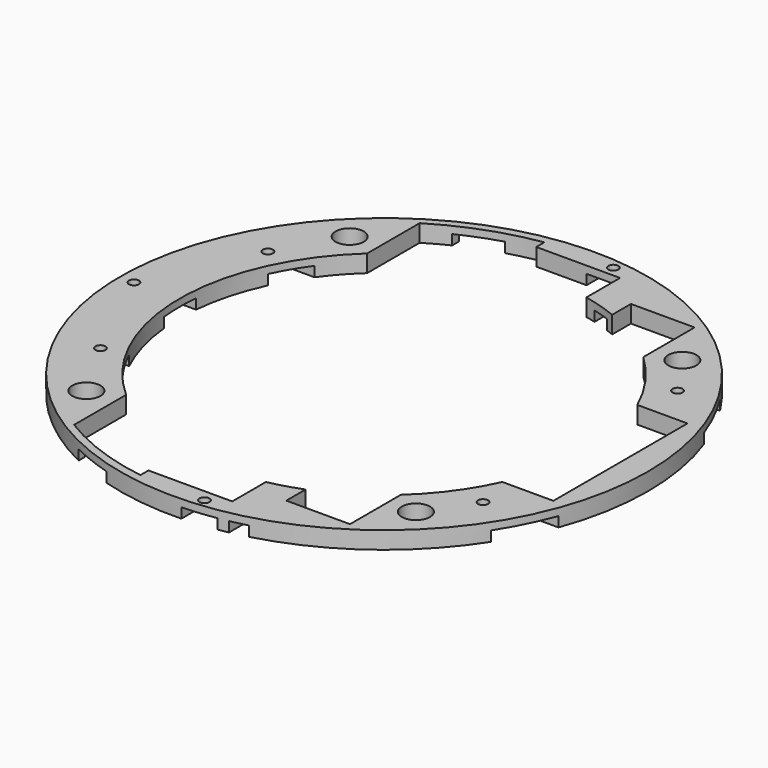
from build123d import *

# Parameters (mm, degrees)
F0_R     = 78.74
F0_R_2   = 4.208
F0_R_3   = 4.2080161266
F1_DEPTH = 5.17
F3_DEPTH = 3
F4_R     = 1.5
F5_DEPTH = 25


# Not quite as in the source:
# - a feature names something its author has since deleted; it is built from what else it names


with BuildPart() as f1:
    # F0 (on Top) → F1 (new body)
    with BuildSketch(Plane.XY):
        with Locations((-0.1257307514, 0.2739626218)):
            Circle(F0_R)
        with Locations((-49.0250116127, -49.6047185081)):
            Circle(F0_R_2, mode=Mode.SUBTRACT)
        with Locations((49.0554707364, -49.3247707953)):
            Circle(F0_R_3, mode=Mode.SUBTRACT)
        with Locations((-49.7306512766, 49.450932452)):
            Circle(F0_R_2, mode=Mode.SUBTRACT)
        with BuildLine():
            ThreePointArc((41.6625381497, 44.7120159348), (49.6362217188, 35.5549502263), (55.6382636856, 25))
            Line((55.6382636856, 25), (70.6142692486, 25))
            Line((70.6142692486, 25), (70.6142692486, -25))
            Line((70.6142692486, -25), (55.3920755218, -25))
            ThreePointArc((55.3920755218, -25), (49.182592498, -35.6382812281), (40.9624707364, -44.8121738117))
            Line((40.9624707364, -44.8121738117), (40.9624707364, -63.790228106))
            Line((40.9624707364, -63.790228106), (21.9624707364, -63.790228106))
            Line((21.9624707364, -63.790228106), (21.9624707364, -56.5864924857))
            ThreePointArc((21.9624707364, -56.5864924857), (17.2267771251, -58.2058669812), (12.3742692486, -59.4315647605))
            Line((12.3742692486, -59.4315647605), (12.3742692486, -71.9660373782))
            Line((12.3742692486, -71.9660373782), (-12.6257307514, -71.9660373782))
            Line((-12.6257307514, -71.9660373782), (-12.6257307514, -74.9675166541))
            ThreePointArc((-12.6257307514, -74.9675166541), (-27.09160778, -71.308076376), (-40.5250116127, -64.8121728344))
            Line((-40.5250116127, -64.8121728344), (-40.5250116127, -45.4305022137))
            ThreePointArc((-40.5250116127, -45.4305022137), (-61.1238878157, -0.2002048119), (-41.2306512766, 45.3448568731))
            Line((-41.2306512766, 45.3448568731), (-41.2306512766, 64.9332740284))
            ThreePointArc((-41.2306512766, 64.9332740284), (-27.3884909599, 71.6521165865), (-12.5, 75.5355537871))
            Line((-12.5, 75.5355537871), (-12.5, 72.5138622393))
            Line((-12.5, 72.5138622393), (0, 72.5138622393))
            Line((0, 72.5138622393), (12.5, 72.5138622393))
            Line((12.5, 72.5138622393), (12.5, 59.9530286583))
            ThreePointArc((12.5, 59.9530286583), (17.6487859305, 58.6269107626), (22.6625381497, 56.8574831953))
            Line((22.6625381497, 56.8574831953), (22.6625381497, 63.8574831953))
            Line((22.6625381497, 63.8574831953), (41.6625381497, 63.8574831953))
            Line((41.6625381497, 63.8574831953), (41.6625381497, 44.7120159348))
        make_face(mode=Mode.SUBTRACT)
        with Locations((49.75511293, 49.1690173001)):
            Circle(F0_R_2, mode=Mode.SUBTRACT)
    extrude(amount=F1_DEPTH)

    # F2 (on face) → F3 (cut)
    with BuildSketch(Plane(origin=(0, 0, 0), x_dir=(1, 0, 0), z_dir=(0, 0, -1))):
        with BuildLine():
            ThreePointArc((-22.6257307514, 75.1828965761), (-28.7215245435, 73.0899806842), (-34.6257307514, 70.5055372352))
            Line((-34.6257307514, 70.5055372352), (-34.6257307514, 68.081065471))
            ThreePointArc((-34.6257307514, 68.081065471), (-28.7284061022, 70.69020135), (-22.6257307514, 72.7742794712))
            Line((-22.6257307514, 72.7742794712), (-22.6257307514, 75.1828965761))
        make_face()
        with BuildLine():
            Line((-34.5, -68.6212157755), (-34.5, -71.1146092424))
            ThreePointArc((-34.5, -71.1146092424), (-28.5952430236, -73.6870028189), (-22.5, -75.7681986639))
            Line((-22.5, -75.7681986639), (-22.5, -73.2755617719))
            ThreePointArc((-22.5, -73.2755617719), (-28.595756362, -71.1952712241), (-34.5, -68.6212157755))
        make_face()
        with BuildLine():
            ThreePointArc((-49.5286609465, -36.0559481471), (-52.707319331, -31.1960670528), (-55.4094464584, -26.0559481471))
            Line((-55.4094464584, -26.0559481471), (-74.5251717599, -26.0559481471))
            ThreePointArc((-74.5251717599, -26.0559481471), (-72.5682702123, -31.1295306193), (-70.2658555864, -36.0559481471))
            Line((-70.2658555864, -36.0559481471), (-49.5286609465, -36.0559481471))
        make_face()
        with BuildLine():
            ThreePointArc((-60.8510849569, -6.0559481471), (-61.1253373513, -0.0548857934), (-60.807987598, 5.9440518529))
            Line((-60.807987598, 5.9440518529), (-78.6198317781, 5.9440518529))
            ThreePointArc((-78.6198317781, 5.9440518529), (-78.86542717, -0.0553124259), (-78.6531542631, -6.0559481471))
            Line((-78.6531542631, -6.0559481471), (-60.8510849569, -6.0559481471))
        make_face()
        with BuildLine():
            ThreePointArc((-55.2039997602, 25.9440518529), (-52.4464078958, 31.0875861785), (-49.2098975215, 35.9440518529))
            Line((-49.2098975215, 35.9440518529), (-70.0417019419, 35.9440518529))
            ThreePointArc((-70.0417019419, 35.9440518529), (-72.3803771023, 31.0190666452), (-74.3726385456, 25.9440518529))
            Line((-74.3726385456, 25.9440518529), (-55.2039997602, 25.9440518529))
        make_face()
        with BuildLine():
            Line((2.5, -72.5138622393), (2.5, -78.9701705229))
            ThreePointArc((2.5, -78.9701705229), (7.5155682015, -78.6423117834), (12.5, -77.9951214075))
            Line((12.5, -77.9951214075), (12.5, -72.5138622393))
            Line((12.5, -72.5138622393), (2.5, -72.5138622393))
        make_face()
        with BuildLine():
            ThreePointArc((12.3742692486, 77.4675166541), (7.3895759923, 78.1065691737), (2.3742692486, 78.4263397919))
            Line((2.3742692486, 78.4263397919), (2.3742692486, 71.9660373782))
            Line((2.3742692486, 71.9660373782), (12.3742692486, 71.9660373782))
            Line((12.3742692486, 71.9660373782), (12.3742692486, 77.4675166541))
        make_face()
        with BuildLine():
            ThreePointArc((20.3742692486, 75.7506228753), (17.8838503139, 76.3787776414), (15.3742692486, 76.9253741629))
            Line((15.3742692486, 76.9253741629), (15.3742692486, 58.7239186961))
            ThreePointArc((15.3742692486, 58.7239186961), (17.8908537815, 58.0047014138), (20.3742692486, 57.1781913848))
            Line((20.3742692486, 57.1781913848), (20.3742692486, 75.7506228753))
        make_face()
        with BuildLine():
            Line((15.5, -59.238668493), (15.5, -77.4479487731))
            ThreePointArc((15.5, -77.4479487731), (18.0096554679, -76.8970359527), (20.5, -76.2645332932))
            Line((20.5, -76.2645332932), (20.5, -57.6810983365))
            ThreePointArc((20.5, -57.6810983365), (18.0167228167, -58.5135658015), (15.5, -59.238668493))
        make_face()
        with BuildLine():
            ThreePointArc((66.3344029178, -42.5), (70.5632346959, -34.9590857149), (73.9398248467, -27))
            Line((73.9398248467, -27), (54.7078258181, -27))
            ThreePointArc((54.7078258181, -27), (49.9060787318, -35.1712123678), (43.8965564147, -42.5))
            Line((43.8965564147, -42.5), (66.3344029178, -42.5))
        make_face()
        with BuildLine():
            ThreePointArc((73.7398130624, 27), (70.2892388263, 34.9640801641), (65.9830865246, 42.5))
            Line((65.9830865246, 42.5), (43.3643614724, 42.5))
            ThreePointArc((43.3643614724, 42.5), (49.5096317795, 35.1848978566), (54.4373608299, 27))
            Line((54.4373608299, 27), (73.7398130624, 27))
        make_face()
    extrude(amount=-F3_DEPTH, mode=Mode.SUBTRACT)

    # F4 (on face) → F5 (cut)
    with BuildSketch(Plane(origin=(0, 0, 3), x_dir=(1, 0, 0), z_dir=(0, 0, -1))):
        with Locations((-74.5251700282, 0)):
            Circle(F4_R)
        with Locations((-59.8972582664, 30.7893175632)):
            Circle(F4_R)
        with Locations((-59.8972582664, -31.6777378321)):
            Circle(F4_R)
        with Locations((8.0563814701, -75.5707131466)):
            Circle(F4_R)
        with Locations((6.9561954952, 75.5563961955)):
            Circle(F4_R)
        with Locations((58.2362919726, 35.7437855263)):
            Circle(F4_R)
        with Locations((58.4940314293, -36.4654541612)):
            Circle(F4_R)
    extrude(amount=-F5_DEPTH, mode=Mode.SUBTRACT)


solid = f1.part
